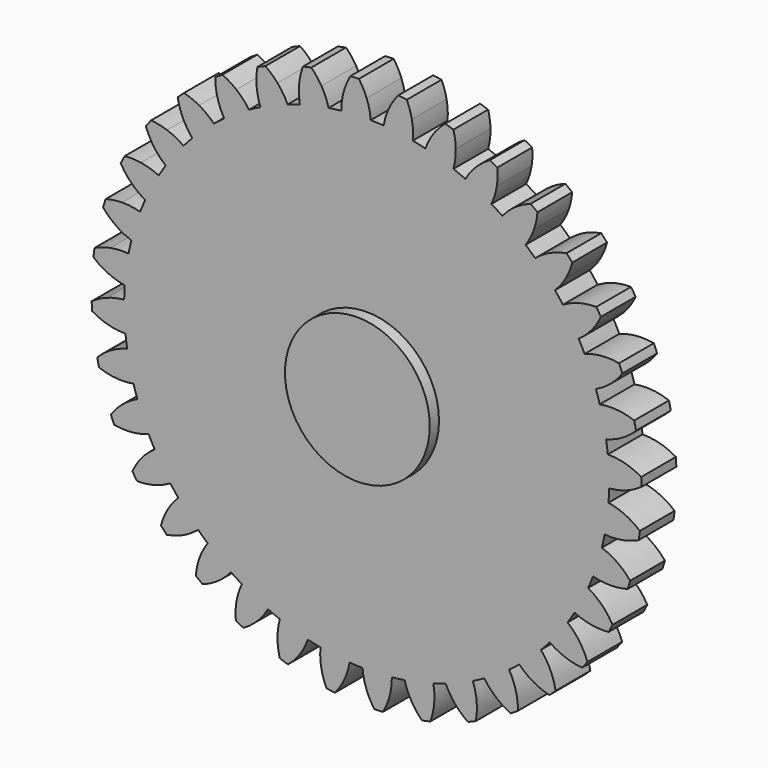
from build123d import *

# Parameters (mm, degrees)
F0_R     = 25
F1_DEPTH = 15
F2_COUNT = 36
F4_DEPTH = 4
F5_DEPTH = 23


with BuildPart() as f1:
    # F0 (on Front) → F1 (new body)
    with BuildSketch(Plane.XZ):
        with BuildLine():
            ThreePointArc((-8.7190556623, 83.2949012146), (-3.6531236918, 83.6702885575), (1.4262480407, 83.7378547404))
            ThreePointArc((1.4262480407, 83.7378547404), (0.9377107983, 86.9200786033), (0, 90))
            ThreePointArc((0, 90), (-1.1760420962, 92.5650071018), (-2.663884374, 94.9626438135))
            ThreePointArc((-2.663884374, 94.9626438135), (-4.1438417997, 94.9095810503), (-5.6227922652, 94.833455105))
            ThreePointArc((-5.6227922652, 94.833455105), (-6.8960050455, 92.3152681261), (-7.8440168473, 89.6575228283))
            ThreePointArc((-7.8440168473, 89.6575228283), (-8.509726536, 86.5075945813), (-8.7190556623, 83.2949012146))
        make_face()
        with BuildLine():
            ThreePointArc((-8.7190556623, 83.2949012146), (-56.0528393049, -62.2265353837), (83.75, 0))
            ThreePointArc((83.75, 0), (59.7223189997, 58.7137727735), (1.4262480407, 83.7378547404))
            ThreePointArc((1.4262480407, 83.7378547404), (-3.6531236918, 83.6702885575), (-8.7190556623, 83.2949012146))
        make_face()
        Circle(F0_R, mode=Mode.SUBTRACT)
        Circle(F0_R)
    extrude(amount=F1_DEPTH)


with BuildPart() as f2_1:
    # F2: instance of F1
    add(f1.part.rotate(Axis((0, 0, 0), (0, 1, 0)), 1 * 360 / F2_COUNT))


with BuildPart() as f2_2:
    # F2: instance of F1
    add(f1.part.rotate(Axis((0, 0, 0), (0, 1, 0)), 2 * 360 / F2_COUNT))


with BuildPart() as f2_3:
    # F2: instance of F1
    add(f1.part.rotate(Axis((0, 0, 0), (0, 1, 0)), 3 * 360 / F2_COUNT))


with BuildPart() as f2_4:
    # F2: instance of F1
    add(f1.part.rotate(Axis((0, 0, 0), (0, 1, 0)), 4 * 360 / F2_COUNT))


with BuildPart() as f2_5:
    # F2: instance of F1
    add(f1.part.rotate(Axis((0, 0, 0), (0, 1, 0)), 5 * 360 / F2_COUNT))


with BuildPart() as f2_6:
    # F2: instance of F1
    add(f1.part.rotate(Axis((0, 0, 0), (0, 1, 0)), 6 * 360 / F2_COUNT))


with BuildPart() as f2_7:
    # F2: instance of F1
    add(f1.part.rotate(Axis((0, 0, 0), (0, 1, 0)), 7 * 360 / F2_COUNT))


with BuildPart() as f2_8:
    # F2: instance of F1
    add(f1.part.rotate(Axis((0, 0, 0), (0, 1, 0)), 8 * 360 / F2_COUNT))


with BuildPart() as f2_9:
    # F2: instance of F1
    add(f1.part.rotate(Axis((0, 0, 0), (0, 1, 0)), 9 * 360 / F2_COUNT))


with BuildPart() as f2_10:
    # F2: instance of F1
    add(f1.part.rotate(Axis((0, 0, 0), (0, 1, 0)), 10 * 360 / F2_COUNT))


with BuildPart() as f2_11:
    # F2: instance of F1
    add(f1.part.rotate(Axis((0, 0, 0), (0, 1, 0)), 11 * 360 / F2_COUNT))


with BuildPart() as f2_12:
    # F2: instance of F1
    add(f1.part.rotate(Axis((0, 0, 0), (0, 1, 0)), 12 * 360 / F2_COUNT))


with BuildPart() as f2_13:
    # F2: instance of F1
    add(f1.part.rotate(Axis((0, 0, 0), (0, 1, 0)), 13 * 360 / F2_COUNT))


with BuildPart() as f2_14:
    # F2: instance of F1
    add(f1.part.rotate(Axis((0, 0, 0), (0, 1, 0)), 14 * 360 / F2_COUNT))


with BuildPart() as f2_15:
    # F2: instance of F1
    add(f1.part.rotate(Axis((0, 0, 0), (0, 1, 0)), 15 * 360 / F2_COUNT))


with BuildPart() as f2_16:
    # F2: instance of F1
    add(f1.part.rotate(Axis((0, 0, 0), (0, 1, 0)), 16 * 360 / F2_COUNT))


with BuildPart() as f2_17:
    # F2: instance of F1
    add(f1.part.rotate(Axis((0, 0, 0), (0, 1, 0)), 17 * 360 / F2_COUNT))


with BuildPart() as f2_18:
    # F2: instance of F1
    add(f1.part.rotate(Axis((0, 0, 0), (0, 1, 0)), 18 * 360 / F2_COUNT))


with BuildPart() as f2_19:
    # F2: instance of F1
    add(f1.part.rotate(Axis((0, 0, 0), (0, 1, 0)), 19 * 360 / F2_COUNT))


with BuildPart() as f2_20:
    # F2: instance of F1
    add(f1.part.rotate(Axis((0, 0, 0), (0, 1, 0)), 20 * 360 / F2_COUNT))


with BuildPart() as f2_21:
    # F2: instance of F1
    add(f1.part.rotate(Axis((0, 0, 0), (0, 1, 0)), 21 * 360 / F2_COUNT))


with BuildPart() as f2_22:
    # F2: instance of F1
    add(f1.part.rotate(Axis((0, 0, 0), (0, 1, 0)), 22 * 360 / F2_COUNT))


with BuildPart() as f2_23:
    # F2: instance of F1
    add(f1.part.rotate(Axis((0, 0, 0), (0, 1, 0)), 23 * 360 / F2_COUNT))


with BuildPart() as f2_24:
    # F2: instance of F1
    add(f1.part.rotate(Axis((0, 0, 0), (0, 1, 0)), 24 * 360 / F2_COUNT))


with BuildPart() as f2_25:
    # F2: instance of F1
    add(f1.part.rotate(Axis((0, 0, 0), (0, 1, 0)), 25 * 360 / F2_COUNT))


with BuildPart() as f2_26:
    # F2: instance of F1
    add(f1.part.rotate(Axis((0, 0, 0), (0, 1, 0)), 26 * 360 / F2_COUNT))


with BuildPart() as f2_27:
    # F2: instance of F1
    add(f1.part.rotate(Axis((0, 0, 0), (0, 1, 0)), 27 * 360 / F2_COUNT))


with BuildPart() as f2_28:
    # F2: instance of F1
    add(f1.part.rotate(Axis((0, 0, 0), (0, 1, 0)), 28 * 360 / F2_COUNT))


with BuildPart() as f2_29:
    # F2: instance of F1
    add(f1.part.rotate(Axis((0, 0, 0), (0, 1, 0)), 29 * 360 / F2_COUNT))


with BuildPart() as f2_30:
    # F2: instance of F1
    add(f1.part.rotate(Axis((0, 0, 0), (0, 1, 0)), 30 * 360 / F2_COUNT))


with BuildPart() as f2_31:
    # F2: instance of F1
    add(f1.part.rotate(Axis((0, 0, 0), (0, 1, 0)), 31 * 360 / F2_COUNT))


with BuildPart() as f2_32:
    # F2: instance of F1
    add(f1.part.rotate(Axis((0, 0, 0), (0, 1, 0)), 32 * 360 / F2_COUNT))


with BuildPart() as f2_33:
    # F2: instance of F1
    add(f1.part.rotate(Axis((0, 0, 0), (0, 1, 0)), 33 * 360 / F2_COUNT))


with BuildPart() as f2_34:
    # F2: instance of F1
    add(f1.part.rotate(Axis((0, 0, 0), (0, 1, 0)), 34 * 360 / F2_COUNT))


with BuildPart() as f2_35:
    # F2: instance of F1
    add(f1.part.rotate(Axis((0, 0, 0), (0, 1, 0)), 35 * 360 / F2_COUNT))


with BuildPart() as f2_11_1:
    add(f2_11.part)

    # F3: union F2_1, F2_22, F2_28, F2_32, F2_31, F2_10, F2_17, F2_23, F2_18, F2_29, F2_30, F2_15, F2_33, F2_12, F2_21, F2_34, F2_16, F1, F2_24, F2_27, F2_20, F2_14, F2_25, F2_26, F2_35, F2_9, F2_19, F2_6, F2_3, F2_13, F2_7, F2_5, F2_8, F2_4, F2_2
    add(f2_1.part)
    add(f2_22.part)
    add(f2_28.part)
    add(f2_32.part)
    add(f2_31.part)
    add(f2_10.part)
    add(f2_17.part)
    add(f2_23.part)
    add(f2_18.part)
    add(f2_29.part)
    add(f2_30.part)
    add(f2_15.part)
    add(f2_33.part)
    add(f2_12.part)
    add(f2_21.part)
    add(f2_34.part)
    add(f2_16.part)
    add(f1.part)
    add(f2_24.part)
    add(f2_27.part)
    add(f2_20.part)
    add(f2_14.part)
    add(f2_25.part)
    add(f2_26.part)
    add(f2_35.part)
    add(f2_9.part)
    add(f2_19.part)
    add(f2_6.part)
    add(f2_3.part)
    add(f2_13.part)
    add(f2_7.part)
    add(f2_5.part)
    add(f2_8.part)
    add(f2_4.part)
    add(f2_2.part)

    # F0 (on Front) → F4 (join)
    with BuildSketch(Plane.XZ):
        Circle(F0_R)
    extrude(amount=-F4_DEPTH)

    # F5 (add): a face of the model
    f5_faces = [f2_11_1.faces().sort_by_distance(p)[0] for p in [
        (0, 4, 0),
    ]]
    extrude(f5_faces, amount=-F5_DEPTH)


solid = f2_11_1.part
